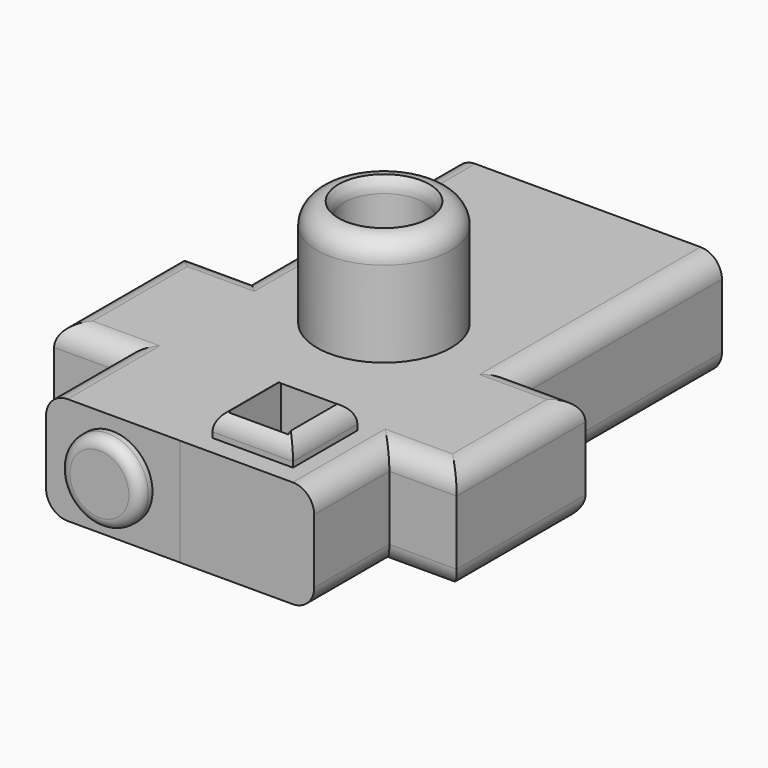
from build123d import *

# Parameters (mm, degrees)
F0_W        = 19.05
F0_H        = 19.05
F0_R        = 15.875
F1_DEPTH    = 25.4
F0_R_2      = 9.525
F2_DEPTH    = 50.8
F0_W_2      = 13.97
F0_H_2      = 15.24
F3_DEPTH    = 31.75
F4_R        = 9.525
F5_DEPTH    = 3.81
F6_R        = 2.54
F7_R        = 5.08
F9_T1_DEPTH = 44.45
F9_T3_DEPTH = 44.45
F10_R       = 5.08
F11_SIZE    = 5.08
F12_SIZE    = 5.08


# Not quite as in the source:
# - a fillet or chamfer that OpenCascade refuses, or shapes differently, is made with other operations: its cross-section is extruded or revolved along the edge and cut away or added


with BuildPart() as f1:
    # F0 (on Top) → F1 (new body)
    with BuildSketch(Plane.XY):
        Polygon((31.75, 60.325), (0, 60.325), (-31.75, 60.325), (-31.75, 0), (-47.625, 0), (-47.625, -38.1), (-31.75, -38.1), (-31.75, -60.325), (0, -60.325), (0, -60.3444650769), (31.75, -60.3444650769), (31.75, -38.1), (47.7005839348, -38.1), (47.7005839348, 0), (47.625, 0), (31.75, 0), align=None)
        with Locations((13.5087583899, -46.2022918522)):
            Rectangle(F0_W, F0_H, mode=Mode.SUBTRACT)
        Circle(F0_R, mode=Mode.SUBTRACT)
    extrude(amount=F1_DEPTH)

    # F0 (on Top) → F2 (join)
    with BuildSketch(Plane.XY):
        Circle(F0_R)
        Circle(F0_R_2, mode=Mode.SUBTRACT)
    extrude(amount=F2_DEPTH)

    # F0 (on Top) → F3 (join)
    with BuildSketch(Plane.XY):
        with Locations((13.5087583899, -46.2022918522)):
            Rectangle(F0_W, F0_H)
        with Locations((13.3824522054, -46.1642474878)):
            Rectangle(F0_W_2, F0_H_2, mode=Mode.SUBTRACT)
    extrude(amount=F3_DEPTH)

    # F4 (on face) → F5 (join)
    with BuildSketch(Plane.XZ.offset(60.325)):
        with Locations((-16.0763879821, 12.6689534055)):
            Circle(F4_R)
    extrude(amount=F5_DEPTH)

    # F6
    f6_edges = [f1.edges().sort_by_distance(p)[0] for p in [
        (-25.601388, -64.135, 12.668953),
    ]]
    fillet(f6_edges, radius=F6_R)

    # F7
    f7_edges = [f1.edges().sort_by_distance(p)[0] for p in [
        (-15.875, 0, 50.8),
    ]]
    fillet(f7_edges, radius=F7_R)

    # F8: fillet of radius 5.08 on 1 edges, made by hand

    # F8_s1 → F8_t2 (revolve, cut)
    with BuildSketch(Plane.XZ):
        with BuildLine():
            ThreePointArc((10.795, 50.8), (9.8530951188, 49.2359470592), (9.525, 47.4398958349))
            Line((9.525, 47.4398958349), (9.525, 50.8))
            Line((9.525, 50.8), (10.795, 50.8))
        make_face()
    revolve(axis=Axis((0, 0, 50.8), (0, 0, 1)), mode=Mode.SUBTRACT)

    # F9: fillet of radius 5.08 on 4 edges, made by hand

    # F9_s2 → F9_t1 (cut)
    with BuildSketch(Plane.XZ.offset(23.9772918522)):
        with BuildLine():
            ThreePointArc((3.9837583899, 26.67), (5.4716559415, 30.2621024484), (9.0637583899, 31.75))
            Line((9.0637583899, 31.75), (3.9837583899, 31.75))
            Line((3.9837583899, 31.75), (3.9837583899, 26.67))
        make_face()
        with BuildLine():
            ThreePointArc((23.0337583899, 26.67), (21.5458608384, 30.2621024484), (17.9537583899, 31.75))
            Line((17.9537583899, 31.75), (23.0337583899, 31.75))
            Line((23.0337583899, 31.75), (23.0337583899, 26.67))
        make_face()
    extrude(amount=F9_T1_DEPTH, mode=Mode.SUBTRACT)

    # F9_s4 → F9_t3 (cut)
    with BuildSketch(Plane.YZ.offset(-8.7162416101)):
        with BuildLine():
            ThreePointArc((-36.6772918522, 26.67), (-38.1651894038, 30.2621024484), (-41.7572918522, 31.75))
            Line((-41.7572918522, 31.75), (-36.6772918522, 31.75))
            Line((-36.6772918522, 31.75), (-36.6772918522, 26.67))
        make_face()
        with BuildLine():
            ThreePointArc((-55.7272918522, 26.67), (-54.2393943007, 30.2621024484), (-50.6472918522, 31.75))
            Line((-50.6472918522, 31.75), (-55.7272918522, 31.75))
            Line((-55.7272918522, 31.75), (-55.7272918522, 26.67))
        make_face()
    extrude(amount=F9_T3_DEPTH, mode=Mode.SUBTRACT)

    # F10
    f10_edges = [f1.edges().sort_by_distance(p)[0] for p in [
        (39.725292, -38.1, 25.4),
        (31.75, -49.222233, 25.4),
        (-31.75, -49.2125, 25.4),
        (-39.6875, -38.1, 25.4),
        (-31.75, 30.1625, 25.4),
        (-39.6875, 0, 25.4),
        (39.725292, 0, 25.4),
        (31.75, 30.1625, 25.4),
        (-31.75, -49.2125, 0),
        (-31.75, 30.1625, 0),
        (-39.6875, 0, 0),
        (-39.6875, -38.1, 0),
        (-47.625, -19.05, 0),
        (31.75, 30.1625, 0),
        (31.75, -49.222233, 0),
        (39.725292, -38.1, 0),
        (47.700584, -19.05, 0),
        (39.725292, 0, 0),
        (47.700584, -19.05, 25.4),
        (-47.625, -19.05, 25.4),
    ]]
    fillet(f10_edges, radius=F10_R)

    # F11
    f11_edges = [f1.edges().sort_by_distance(p)[0] for p in [
        (13.382452, -38.544247, 0),
        (20.367452, -46.164247, 0),
        (13.382452, -53.784247, 0),
        (6.397452, -46.164247, 0),
    ]]
    chamfer(f11_edges, length=F11_SIZE)

    # F12
    f12_edges = [f1.edges().sort_by_distance(p)[0] for p in [
        (-9.525, 0, 0),
    ]]
    chamfer(f12_edges, length=F12_SIZE)


solid = f1.part
